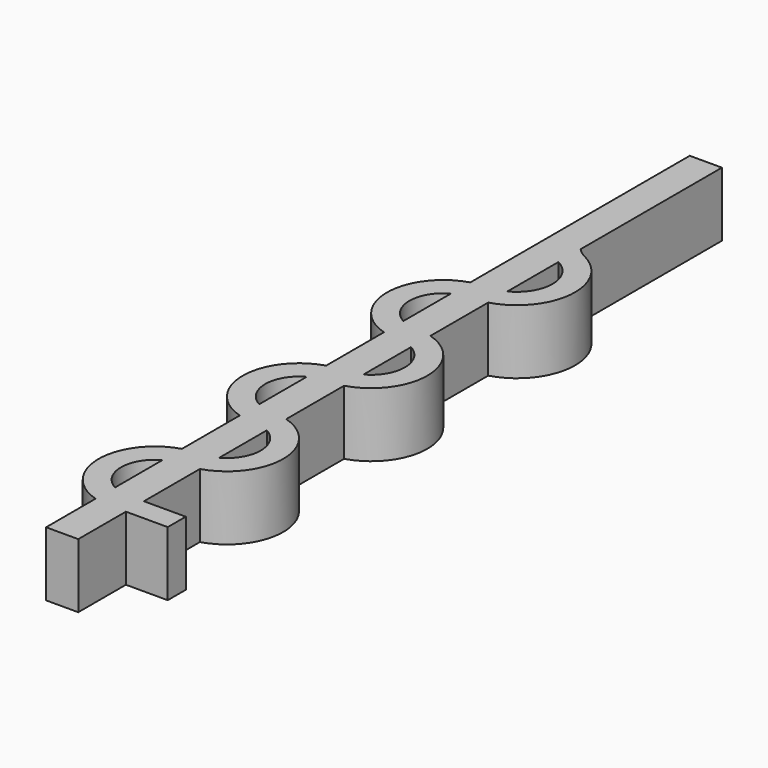
from build123d import *

# Parameters (mm, degrees)
F0_W     = 8.255
F0_H     = 4.445
F1_DEPTH = 12.7


with BuildPart() as f1:
    # F0 (on Top) → F1 (new body)
    with BuildSketch(Plane.XY):
        with BuildLine():
            Line((3.175, 89.2175), (-3.175, 89.2175))
            Line((-3.175, 89.2175), (-3.175, 59.21375))
            ThreePointArc((-3.175, 59.21375), (-1.4603208006, 53.1557160458), (3.175, 48.895))
            Line((3.175, 48.895), (3.175, 54.3686230183))
            Line((3.175, 54.3686230183), (3.175, 89.2175))
        make_face()
        with BuildLine():
            ThreePointArc((3.175, 48.895), (-1.4603208006, 53.1557160458), (-3.175, 59.21375))
            Line((-3.175, 59.21375), (-3.175, 35.0967737428))
            ThreePointArc((-3.175, 35.0967737428), (-1.6043069816, 35.4435836373), (0, 35.56))
            ThreePointArc((0, 35.56), (1.6318769104, 35.751593167), (3.175, 36.315952381))
            Line((3.175, 36.315952381), (3.175, 48.895))
        make_face()
        with BuildLine():
            ThreePointArc((5.178111588, 52.8630686695), (4.1097442392, 53.5269543338), (3.175, 54.3686230183))
            Line((3.175, 54.3686230183), (3.175, 48.895))
            ThreePointArc((3.175, 48.895), (7.0454761905, 42.6054761905), (3.175, 36.315952381))
            Line((3.175, 36.315952381), (3.175, 31.5623598693))
            ThreePointArc((3.175, 31.5623598693), (11.4400029348, 41.5296621103), (5.178111588, 52.8630686695))
        make_face()
        with BuildLine():
            ThreePointArc((0, 35.56), (-1.6043069816, 35.4435836373), (-3.175, 35.0967737428))
            Line((-3.175, 35.0967737428), (-3.175, 30.3105138368))
            ThreePointArc((-3.175, 30.3105138368), (-1.6376677767, 30.9107499954), (0, 31.115))
            ThreePointArc((0, 31.115), (1.6031808891, 31.2273896149), (3.175, 31.5623598693))
            Line((3.175, 31.5623598693), (3.175, 36.315952381))
            ThreePointArc((3.175, 36.315952381), (1.6318769104, 35.751593167), (0, 35.56))
        make_face()
        with BuildLine():
            Line((-3.175, 30.3105138368), (-3.175, 35.0967737428))
            ThreePointArc((-3.175, 35.0967737428), (-11.1125, 24.4475), (-3.175, 13.7982262572))
            Line((-3.175, 13.7982262572), (-3.175, 18.5844861632))
            ThreePointArc((-3.175, 18.5844861632), (-6.6675, 24.4475), (-3.175, 30.3105138368))
        make_face()
        with BuildLine():
            ThreePointArc((0, 31.115), (-1.6376677767, 30.9107499954), (-3.175, 30.3105138368))
            Line((-3.175, 30.3105138368), (-3.175, 18.5844861632))
            ThreePointArc((-3.175, 18.5844861632), (-1.6376677767, 17.9842500046), (0, 17.78))
            ThreePointArc((0, 17.78), (1.6043069816, 17.6635836373), (3.175, 17.3167737428))
            Line((3.175, 17.3167737428), (3.175, 31.5623598693))
            ThreePointArc((3.175, 31.5623598693), (1.6031808891, 31.2273896149), (0, 31.115))
        make_face()
        with BuildLine():
            ThreePointArc((0, 13.335), (-1.6043069816, 13.4514163627), (-3.175, 13.7982262572))
            Line((-3.175, 13.7982262572), (-3.175, -0.4632262572))
            ThreePointArc((-3.175, -0.4632262572), (-1.6043069816, -0.1164163627), (0, 0))
            ThreePointArc((0, 0), (1.6376677767, 0.2042500046), (3.175, 0.8044861632))
            Line((3.175, 0.8044861632), (3.175, 12.5305138368))
            ThreePointArc((3.175, 12.5305138368), (1.6376677767, 13.1307499954), (0, 13.335))
        make_face()
        with BuildLine():
            Line((-3.175, 18.5844861632), (-3.175, 13.7982262572))
            ThreePointArc((-3.175, 13.7982262572), (-1.6043069816, 13.4514163627), (0, 13.335))
            ThreePointArc((0, 13.335), (1.6376677767, 13.1307499954), (3.175, 12.5305138368))
            Line((3.175, 12.5305138368), (3.175, 17.3167737428))
            ThreePointArc((3.175, 17.3167737428), (1.6043069816, 17.6635836373), (0, 17.78))
            ThreePointArc((0, 17.78), (-1.6376677767, 17.9842500046), (-3.175, 18.5844861632))
        make_face()
        with BuildLine():
            ThreePointArc((0, 0), (-1.6043069816, -0.1164163627), (-3.175, -0.4632262572))
            Line((-3.175, -0.4632262572), (-3.175, -5.2494861632))
            ThreePointArc((-3.175, -5.2494861632), (-1.6376677767, -4.6492500046), (0, -4.445))
            ThreePointArc((0, -4.445), (1.6043069816, -4.3285836373), (3.175, -3.9817737428))
            Line((3.175, -3.9817737428), (3.175, 0.8044861632))
            ThreePointArc((3.175, 0.8044861632), (1.6376677767, 0.2042500046), (0, 0))
        make_face()
        with BuildLine():
            Line((-3.175, -5.2494861632), (-3.175, -0.4632262572))
            ThreePointArc((-3.175, -0.4632262572), (-11.1125, -11.1125), (-3.175, -21.7617737428))
            Line((-3.175, -21.7617737428), (-3.175, -16.9755138368))
            ThreePointArc((-3.175, -16.9755138368), (-6.6675, -11.1125), (-3.175, -5.2494861632))
        make_face()
        with BuildLine():
            ThreePointArc((3.175, -3.9817737428), (11.1125, 6.6675), (3.175, 17.3167737428))
            Line((3.175, 17.3167737428), (3.175, 12.5305138368))
            ThreePointArc((3.175, 12.5305138368), (6.6675, 6.6675), (3.175, 0.8044861632))
            Line((3.175, 0.8044861632), (3.175, -3.9817737428))
        make_face()
        with BuildLine():
            ThreePointArc((0, -4.445), (-1.6376677767, -4.6492500046), (-3.175, -5.2494861632))
            Line((-3.175, -5.2494861632), (-3.175, -16.9755138368))
            ThreePointArc((-3.175, -16.9755138368), (-1.6376677767, -17.5757499954), (0, -17.78))
            ThreePointArc((0, -17.78), (1.6043069816, -17.8964163627), (3.175, -18.2432262572))
            Line((3.175, -18.2432262572), (3.175, -3.9817737428))
            ThreePointArc((3.175, -3.9817737428), (1.6043069816, -4.3285836373), (0, -4.445))
        make_face()
        with BuildLine():
            ThreePointArc((0, -22.225), (-1.6043069816, -22.1085836373), (-3.175, -21.7617737428))
            Line((-3.175, -21.7617737428), (-3.175, -36.0232262572))
            ThreePointArc((-3.175, -36.0232262572), (-1.6043069816, -35.6764163627), (0, -35.56))
            ThreePointArc((0, -35.56), (1.6376677767, -35.3557499954), (3.175, -34.7555138368))
            Line((3.175, -34.7555138368), (3.175, -23.0294861632))
            ThreePointArc((3.175, -23.0294861632), (1.6376677767, -22.4292500046), (0, -22.225))
        make_face()
        with BuildLine():
            Line((-3.175, -16.9755138368), (-3.175, -21.7617737428))
            ThreePointArc((-3.175, -21.7617737428), (-1.6043069816, -22.1085836373), (0, -22.225))
            ThreePointArc((0, -22.225), (1.6376677767, -22.4292500046), (3.175, -23.0294861632))
            Line((3.175, -23.0294861632), (3.175, -18.2432262572))
            ThreePointArc((3.175, -18.2432262572), (1.6043069816, -17.8964163627), (0, -17.78))
            ThreePointArc((0, -17.78), (-1.6376677767, -17.5757499954), (-3.175, -16.9755138368))
        make_face()
        with BuildLine():
            ThreePointArc((0, -35.56), (-1.6043069816, -35.6764163627), (-3.175, -36.0232262572))
            Line((-3.175, -36.0232262572), (-3.175, -40.8094861632))
            ThreePointArc((-3.175, -40.8094861632), (-1.6376677767, -40.2092500046), (0, -40.005))
            ThreePointArc((0, -40.005), (1.6043069816, -39.8885836373), (3.175, -39.5417737428))
            Line((3.175, -39.5417737428), (3.175, -34.7555138368))
            ThreePointArc((3.175, -34.7555138368), (1.6376677767, -35.3557499954), (0, -35.56))
        make_face()
        with BuildLine():
            Line((-3.175, -40.8094861632), (-3.175, -36.0232262572))
            ThreePointArc((-3.175, -36.0232262572), (-11.1125, -46.6725), (-3.175, -57.3217737428))
            Line((-3.175, -57.3217737428), (-3.175, -52.5355138368))
            ThreePointArc((-3.175, -52.5355138368), (-6.6675, -46.6725), (-3.175, -40.8094861632))
        make_face()
        with BuildLine():
            ThreePointArc((3.175, -39.5417737428), (11.1125, -28.8925), (3.175, -18.2432262572))
            Line((3.175, -18.2432262572), (3.175, -23.0294861632))
            ThreePointArc((3.175, -23.0294861632), (6.6675, -28.8925), (3.175, -34.7555138368))
            Line((3.175, -34.7555138368), (3.175, -39.5417737428))
        make_face()
        with BuildLine():
            ThreePointArc((0, -40.005), (-1.6376677767, -40.2092500046), (-3.175, -40.8094861632))
            Line((-3.175, -40.8094861632), (-3.175, -52.5355138368))
            ThreePointArc((-3.175, -52.5355138368), (-1.6376677767, -53.1357499954), (0, -53.34))
            Line((0, -53.34), (3.175, -53.34))
            Line((3.175, -53.34), (3.175, -39.5417737428))
            ThreePointArc((3.175, -39.5417737428), (1.6043069816, -39.8885836373), (0, -40.005))
        make_face()
        with BuildLine():
            ThreePointArc((0, -57.785), (-1.6043069816, -57.6685836373), (-3.175, -57.3217737428))
            Line((-3.175, -57.3217737428), (-3.175, -69.5325))
            Line((-3.175, -69.5325), (3.175, -69.5325))
            Line((3.175, -69.5325), (3.175, -57.785))
            Line((3.175, -57.785), (0, -57.785))
        make_face()
        with BuildLine():
            Line((-3.175, -52.5355138368), (-3.175, -57.3217737428))
            ThreePointArc((-3.175, -57.3217737428), (-1.6043069816, -57.6685836373), (0, -57.785))
            Line((0, -57.785), (3.175, -57.785))
            Line((3.175, -57.785), (3.175, -53.34))
            Line((3.175, -53.34), (0, -53.34))
            ThreePointArc((0, -53.34), (-1.6376677767, -53.1357499954), (-3.175, -52.5355138368))
        make_face()
        with Locations((7.3025, -55.5625)):
            Rectangle(F0_W, F0_H)
    extrude(amount=F1_DEPTH)


solid = f1.part
